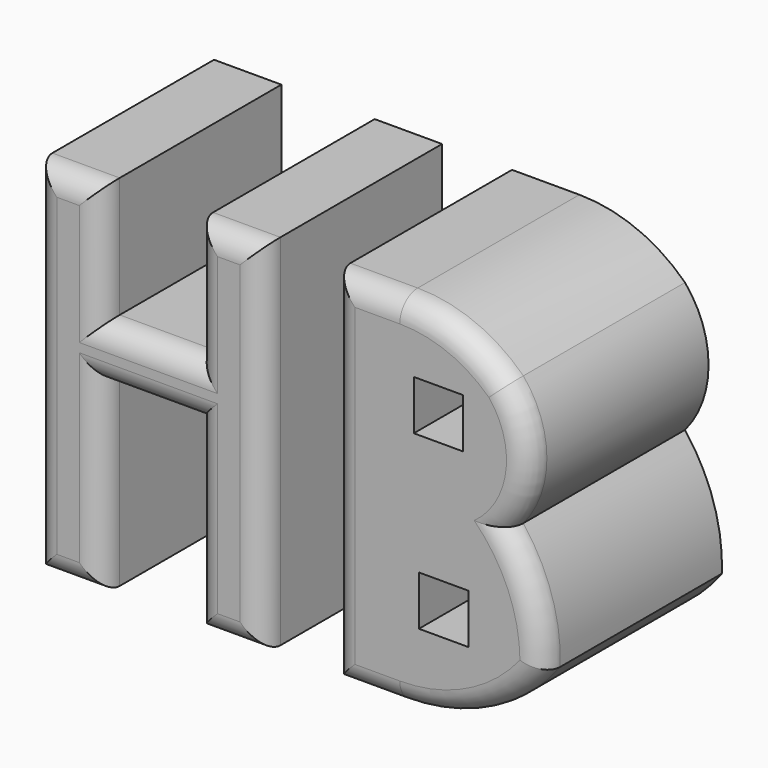
from build123d import *

# Parameters (mm, degrees)
F1_DEPTH       = 50
F0_W           = 11
F0_H           = 11.0476613045
F0_H_2         = 11.0476617701
F2_T1_DEPTH    = 105
F2_T3_DEPTH    = 40
F2_T5_DEPTH    = 39.3571444373
F2_T7_DEPTH    = 40
F2_T9_DEPTH    = 53.6428555627
F2_T11_DEPTH   = 20.7857115482
F2_T16_DEPTH   = 51.8571444373
F2_T21_DEPTH   = 66.1428555627
F2_T26_DEPTH   = 66.1428555627
F2_T31_DEPTH   = 51.8571444373
F2_T37_DEPTH   = 51.8571444373
F2_T42_DEPTH   = 33.2857115482
F2_T49_DEPTH   = 66.1428555627
F2_T54_DEPTH   = 33.2857115482
F2_T61_DEPTH   = 33.2857115482
F2_T65_DEPTH   = 66.1428555627
F2_T73_DEPTH   = 51.8571444373
F2_T78_DEPTH   = 33.2857115482
F2_2_T1_DEPTH  = 27.5
F2_2_T3_DEPTH  = 105
F2_2_T6_ANGLE  = 80.3342530923
F2_2_T10_ANGLE = 143.4118786012
F2_2_S11_R     = 39.2893999544
F2_2_T12_DEPTH = 27
F2_2_T16_ANGLE = 76.3206243735
F2_2_S17_R     = 22.5233307718
F2_2_T18_DEPTH = 29
F2_2_T20_ANGLE = 71.8308511896
F2_2_T25_ANGLE = 76.3206243735
F2_2_S26_R     = 22.5233307718
F2_2_T27_DEPTH = 29
F2_2_T30_ANGLE = 143.4118786012
F2_2_S31_R     = 39.2893999544
F2_2_T32_DEPTH = 27


# Not quite as in the source:
# - a fillet or chamfer that OpenCascade refuses, or shapes differently, is made with other operations: its cross-section is extruded or revolved along the edge and cut away or added


with BuildPart() as f1:
    # F0 (on Front) → F1 (new body)
    with BuildSketch(Plane.XZ):
        Polygon((-35.7857115482, 33.0714304233), (-50.7857115482, 33.0714304233), (-50.7857115482, -46.9285695767), (-35.7857115482, -46.9285695767), (-35.7857115482, -5.785714014), (-15, -5.785714014), (-15, -46.9285695767), (0, -46.9285695767), (0, 33.0714304233), (-15, 33.0714304233), (-15, 6.214285986), (-35.7857115482, 6.214285986), align=None)
    extrude(amount=F1_DEPTH)

    # F2: fillet of radius 5 on 12 edges, made by hand

    # F2_s2 → F2_t1 (cut)
    with BuildSketch(Plane.XY.offset(-59.4285695767)):
        with BuildLine():
            ThreePointArc((0, -45), (-1.4644660941, -48.5355339059), (-5, -50))
            Line((-5, -50), (0, -50))
            Line((0, -50), (0, -45))
        make_face()
        with BuildLine():
            ThreePointArc((-50.7857115482, -45), (-49.3212454541, -48.5355339059), (-45.7857115482, -50))
            Line((-45.7857115482, -50), (-50.7857115482, -50))
            Line((-50.7857115482, -50), (-50.7857115482, -45))
        make_face()
    extrude(amount=F2_T1_DEPTH, mode=Mode.SUBTRACT)

    # F2_s4 → F2_t3 (cut)
    with BuildSketch(Plane.YZ.offset(-27.5)):
        with BuildLine():
            ThreePointArc((-45, 33.0714304233), (-48.5355339059, 31.6069643292), (-50, 28.0714304233))
            Line((-50, 28.0714304233), (-50, 33.0714304233))
            Line((-50, 33.0714304233), (-45, 33.0714304233))
        make_face()
        with BuildLine():
            ThreePointArc((-45, -46.9285695767), (-48.5355339059, -45.4641034826), (-50, -41.9285695767))
            Line((-50, -41.9285695767), (-50, -46.9285695767))
            Line((-50, -46.9285695767), (-45, -46.9285695767))
        make_face()
    extrude(amount=F2_T3_DEPTH, mode=Mode.SUBTRACT)

    # F2_s6 → F2_t5 (cut)
    with BuildSketch(Plane.XY.offset(6.214285986)):
        with BuildLine():
            ThreePointArc((-35.7857115482, -45), (-37.2501776423, -48.5355339059), (-40.7857115482, -50))
            Line((-40.7857115482, -50), (-35.7857115482, -50))
            Line((-35.7857115482, -50), (-35.7857115482, -45))
        make_face()
        with BuildLine():
            ThreePointArc((-15, -45), (-13.5355339059, -48.5355339059), (-10, -50))
            Line((-10, -50), (-15, -50))
            Line((-15, -50), (-15, -45))
        make_face()
    extrude(amount=F2_T5_DEPTH, mode=Mode.SUBTRACT)

    # F2_s8 → F2_t7 (cut)
    with BuildSketch(Plane.YZ.offset(-63.2857115482)):
        with BuildLine():
            ThreePointArc((-45, 33.0714304233), (-48.5355339059, 31.6069643292), (-50, 28.0714304233))
            Line((-50, 28.0714304233), (-50, 33.0714304233))
            Line((-50, 33.0714304233), (-45, 33.0714304233))
        make_face()
        with BuildLine():
            ThreePointArc((-45, -46.9285695767), (-48.5355339059, -45.4641034826), (-50, -41.9285695767))
            Line((-50, -41.9285695767), (-50, -46.9285695767))
            Line((-50, -46.9285695767), (-45, -46.9285695767))
        make_face()
    extrude(amount=F2_T7_DEPTH, mode=Mode.SUBTRACT)

    # F2_s10 → F2_t9 (cut)
    with BuildSketch(Plane.XY.offset(-59.4285695767)):
        with BuildLine():
            ThreePointArc((-35.7857115482, -45), (-37.2501776423, -48.5355339059), (-40.7857115482, -50))
            Line((-40.7857115482, -50), (-35.7857115482, -50))
            Line((-35.7857115482, -50), (-35.7857115482, -45))
        make_face()
        with BuildLine():
            ThreePointArc((-15, -45), (-13.5355339059, -48.5355339059), (-10, -50))
            Line((-10, -50), (-15, -50))
            Line((-15, -50), (-15, -45))
        make_face()
    extrude(amount=F2_T9_DEPTH, mode=Mode.SUBTRACT)

    # F2_s12 → F2_t11 (cut)
    with BuildSketch(Plane.YZ.offset(-35.7857115482)):
        with BuildLine():
            ThreePointArc((-45, -5.785714014), (-48.5355339059, -4.3212479199), (-50, -0.785714014))
            Line((-50, -0.785714014), (-50, -5.785714014))
            Line((-50, -5.785714014), (-45, -5.785714014))
        make_face()
        with BuildLine():
            ThreePointArc((-45, 6.214285986), (-48.5355339059, 4.749819892), (-50, 1.214285986))
            Line((-50, 1.214285986), (-50, 6.214285986))
            Line((-50, 6.214285986), (-45, 6.214285986))
        make_face()
    extrude(amount=F2_T11_DEPTH, mode=Mode.SUBTRACT)


with BuildPart() as f1b:
    # F0 (on Front) → F1, piece 2 (new body)
    with BuildSketch(Plane.XZ):
        with BuildLine():
            Line((30.5800376087, 33.0714304233), (15.5800376087, 33.0714304233))
            Line((15.5800376087, 33.0714304233), (15.5800376087, -46.9285695767))
            Line((15.5800376087, -46.9285695767), (30.5800376087, -46.9285695767))
            ThreePointArc((30.5800376087, -46.9285695767), (48.3641167152, -42.6873971764), (62.3201467097, -30.8767985553))
            ThreePointArc((62.3201467097, -30.8767985553), (60.4523586567, -17.4078220357), (54.1052147746, -5.3821941838))
            ThreePointArc((54.1052147746, -5.3821941838), (59.3488970656, 9.0647493489), (54.1052147746, 23.5116928816))
            ThreePointArc((54.1052147746, 23.5116928816), (43.2767157427, 30.5902254056), (30.5800376087, 33.0714304233))
        make_face()
        with Locations((40.3426289856, -24.7864220291)):
            Rectangle(F0_W, F0_H, mode=Mode.SUBTRACT)
        with Locations((39.2095372379, 13.1722127553)):
            Rectangle(F0_W, F0_H_2, mode=Mode.SUBTRACT)
    extrude(amount=F1_DEPTH)

    # F2#2: fillet of radius 5 on 7 edges, made by hand

    # F2_2_s2 → F2_2_t1 (cut)
    with BuildSketch(Plane.YZ.offset(3.0800376087)):
        with BuildLine():
            ThreePointArc((-45, -46.9285695767), (-48.5355339059, -45.4641034826), (-50, -41.9285695767))
            Line((-50, -41.9285695767), (-50, -46.9285695767))
            Line((-50, -46.9285695767), (-45, -46.9285695767))
        make_face()
        with BuildLine():
            ThreePointArc((-45, 33.0714304233), (-48.5355339059, 31.6069643292), (-50, 28.0714304233))
            Line((-50, 28.0714304233), (-50, 33.0714304233))
            Line((-50, 33.0714304233), (-45, 33.0714304233))
        make_face()
    extrude(amount=F2_2_T1_DEPTH, mode=Mode.SUBTRACT)

    # F2_2_s4 → F2_2_t3 (cut)
    with BuildSketch(Plane.XY.offset(-59.4285695767)):
        with BuildLine():
            ThreePointArc((15.5800376087, -45), (17.0445037028, -48.5355339059), (20.5800376087, -50))
            Line((20.5800376087, -50), (15.5800376087, -50))
            Line((15.5800376087, -50), (15.5800376087, -45))
        make_face()
    extrude(amount=F2_2_T3_DEPTH, mode=Mode.SUBTRACT)

    # F2_2_s5 → F2_2_t6 (revolve, cut)
    with BuildSketch(Plane(origin=(0.9703990257, 0, -5.6975752164), x_dir=(0, 1, 0), z_dir=(0.1679000671, 0, -0.9858040208))):
        with BuildLine():
            ThreePointArc((-45, 63.7619837133), (-48.5355339059, 62.2975176192), (-50, 58.7619837133))
            Line((-50, 58.7619837133), (-50, 63.7619837133))
            Line((-50, 63.7619837133), (-45, 63.7619837133))
        make_face()
    revolve(axis=Axis((30.5800376087, -50, -0.6545238583), (0, -1, 0)), revolution_arc=F2_2_T6_ANGLE, mode=Mode.SUBTRACT)


with BuildPart() as f2_tool14:
    # F2_s15 → F2_t16 (new body)
    with BuildSketch(Plane.XY.offset(-6.285714014)):
        with BuildLine():
            ThreePointArc((-35.7857115482, -45), (-37.2501776423, -48.5355339059), (-40.7857115482, -50))
            Line((-40.7857115482, -50), (-35.7857115482, -50))
            Line((-35.7857115482, -50), (-35.7857115482, -45))
        make_face()
    extrude(amount=F2_T16_DEPTH)

    split(bisect_by=Plane.XY.offset(-5.785714014), keep=Keep.BOTTOM)


with BuildPart() as f1_1:
    add(f1.part)

    # F2_t13: cut F2_tool14
    add(f2_tool14.part, mode=Mode.SUBTRACT)


with BuildPart() as f2_tool19:
    # F2_s20 → F2_t21 (new body)
    with BuildSketch(Plane.XY.offset(-59.4285695767)):
        with BuildLine():
            ThreePointArc((-35.7857115482, -45), (-37.2501776423, -48.5355339059), (-40.7857115482, -50))
            Line((-40.7857115482, -50), (-35.7857115482, -50))
            Line((-35.7857115482, -50), (-35.7857115482, -45))
        make_face()
    extrude(amount=F2_T21_DEPTH)

    split(bisect_by=Plane.XY.offset(6.214285986), keep=Keep.TOP)


with BuildPart() as f1_2:
    add(f1_1.part)

    # F2_t18: cut F2_tool19
    add(f2_tool19.part, mode=Mode.SUBTRACT)


with BuildPart() as f2_tool24:
    # F2_s25 → F2_t26 (new body)
    with BuildSketch(Plane.XY.offset(6.714285986)):
        with BuildLine():
            ThreePointArc((-15, -45), (-13.5355339059, -48.5355339059), (-10, -50))
            Line((-10, -50), (-15, -50))
            Line((-15, -50), (-15, -45))
        make_face()
    extrude(amount=-F2_T26_DEPTH)

    split(bisect_by=Plane.XY.offset(6.214285986), keep=Keep.TOP)


with BuildPart() as f1_3:
    add(f1_2.part)

    # F2_t23: cut F2_tool24
    add(f2_tool24.part, mode=Mode.SUBTRACT)


with BuildPart() as f2_tool29:
    # F2_s30 → F2_t31 (new body)
    with BuildSketch(Plane.XY.offset(45.5714304233)):
        with BuildLine():
            ThreePointArc((-15, -45), (-13.5355339059, -48.5355339059), (-10, -50))
            Line((-10, -50), (-15, -50))
            Line((-15, -50), (-15, -45))
        make_face()
    extrude(amount=-F2_T31_DEPTH)

    split(bisect_by=Plane.XY.offset(-5.785714014), keep=Keep.BOTTOM)


with BuildPart() as f1_4:
    add(f1_3.part)

    # F2_t28: cut F2_tool29
    add(f2_tool29.part, mode=Mode.SUBTRACT)


with BuildPart() as f2_tool35:
    # F2_s36 → F2_t37 (new body)
    with BuildSketch(Plane.XY.offset(-6.285714014)):
        with BuildLine():
            ThreePointArc((-35.7857115482, -45), (-37.2501776423, -48.5355339059), (-40.7857115482, -50))
            Line((-40.7857115482, -50), (-35.7857115482, -50))
            Line((-35.7857115482, -50), (-35.7857115482, -45))
        make_face()
    extrude(amount=F2_T37_DEPTH)

    split(bisect_by=Plane.XY.offset(6.214285986), keep=Keep.BOTTOM)

    split(bisect_by=Plane.XY.offset(-5.785714014), keep=Keep.TOP)


with BuildPart() as f2_tool40:
    # F2_s41 → F2_t42 (new body)
    with BuildSketch(Plane.YZ.offset(-15)):
        with BuildLine():
            ThreePointArc((-45, 6.214285986), (-48.5355339059, 4.749819892), (-50, 1.214285986))
            Line((-50, 1.214285986), (-50, 6.214285986))
            Line((-50, 6.214285986), (-45, 6.214285986))
        make_face()
    extrude(amount=-F2_T42_DEPTH)

    split(bisect_by=Plane.YZ.offset(-35.7857115482), keep=Keep.BOTTOM)


with BuildPart() as f2_tool35_1:
    add(f2_tool35.part)

    # F2_t44: intersect F2_tool40
    add(f2_tool40.part, mode=Mode.INTERSECT)


with BuildPart() as f1_5:
    add(f1_4.part)

    # F2_t33: cut F2_tool35
    add(f2_tool35_1.part, mode=Mode.SUBTRACT)


with BuildPart() as f2_tool47:
    # F2_s48 → F2_t49 (new body)
    with BuildSketch(Plane.XY.offset(-59.4285695767)):
        with BuildLine():
            ThreePointArc((-35.7857115482, -45), (-37.2501776423, -48.5355339059), (-40.7857115482, -50))
            Line((-40.7857115482, -50), (-35.7857115482, -50))
            Line((-35.7857115482, -50), (-35.7857115482, -45))
        make_face()
    extrude(amount=F2_T49_DEPTH)

    split(bisect_by=Plane.XY.offset(6.214285986), keep=Keep.BOTTOM)

    split(bisect_by=Plane.XY.offset(-5.785714014), keep=Keep.TOP)


with BuildPart() as f2_tool52:
    # F2_s53 → F2_t54 (new body)
    with BuildSketch(Plane.YZ.offset(-48.2857115482)):
        with BuildLine():
            ThreePointArc((-45, -5.785714014), (-48.5355339059, -4.3212479199), (-50, -0.785714014))
            Line((-50, -0.785714014), (-50, -5.785714014))
            Line((-50, -5.785714014), (-45, -5.785714014))
        make_face()
    extrude(amount=F2_T54_DEPTH)

    split(bisect_by=Plane.YZ.offset(-35.7857115482), keep=Keep.BOTTOM)


with BuildPart() as f2_tool47_1:
    add(f2_tool47.part)

    # F2_t56: intersect F2_tool52
    add(f2_tool52.part, mode=Mode.INTERSECT)


with BuildPart() as f1_6:
    add(f1_5.part)

    # F2_t45: cut F2_tool47
    add(f2_tool47_1.part, mode=Mode.SUBTRACT)


with BuildPart() as f2_tool59:
    # F2_s60 → F2_t61 (new body)
    with BuildSketch(Plane.YZ.offset(-35.7857115482)):
        with BuildLine():
            ThreePointArc((-45, -5.785714014), (-48.5355339059, -4.3212479199), (-50, -0.785714014))
            Line((-50, -0.785714014), (-50, -5.785714014))
            Line((-50, -5.785714014), (-45, -5.785714014))
        make_face()
    extrude(amount=F2_T61_DEPTH)

    split(bisect_by=Plane.YZ.offset(-15), keep=Keep.TOP)


with BuildPart() as f2_tool63:
    # F2_s64 → F2_t65 (new body)
    with BuildSketch(Plane.XY.offset(6.714285986)):
        with BuildLine():
            ThreePointArc((-15, -45), (-13.5355339059, -48.5355339059), (-10, -50))
            Line((-10, -50), (-15, -50))
            Line((-15, -50), (-15, -45))
        make_face()
    extrude(amount=-F2_T65_DEPTH)

    split(bisect_by=Plane.XY.offset(-5.785714014), keep=Keep.TOP)

    split(bisect_by=Plane.XY.offset(6.214285986), keep=Keep.BOTTOM)


with BuildPart() as f2_tool59_1:
    add(f2_tool59.part)

    # F2_t68: intersect F2_tool63
    add(f2_tool63.part, mode=Mode.INTERSECT)


with BuildPart() as f1_7:
    add(f1_6.part)

    # F2_t57: cut F2_tool59
    add(f2_tool59_1.part, mode=Mode.SUBTRACT)


with BuildPart() as f2_tool71:
    # F2_s72 → F2_t73 (new body)
    with BuildSketch(Plane.XY.offset(45.5714304233)):
        with BuildLine():
            ThreePointArc((-15, -45), (-13.5355339059, -48.5355339059), (-10, -50))
            Line((-10, -50), (-15, -50))
            Line((-15, -50), (-15, -45))
        make_face()
    extrude(amount=-F2_T73_DEPTH)

    split(bisect_by=Plane.XY.offset(-5.785714014), keep=Keep.TOP)

    split(bisect_by=Plane.XY.offset(6.214285986), keep=Keep.BOTTOM)


with BuildPart() as f2_tool76:
    # F2_s77 → F2_t78 (new body)
    with BuildSketch(Plane.YZ.offset(-2.5)):
        with BuildLine():
            ThreePointArc((-45, 6.214285986), (-48.5355339059, 4.749819892), (-50, 1.214285986))
            Line((-50, 1.214285986), (-50, 6.214285986))
            Line((-50, 6.214285986), (-45, 6.214285986))
        make_face()
    extrude(amount=-F2_T78_DEPTH)

    split(bisect_by=Plane.YZ.offset(-15), keep=Keep.TOP)


with BuildPart() as f2_tool71_1:
    add(f2_tool71.part)

    # F2_t80: intersect F2_tool76
    add(f2_tool76.part, mode=Mode.INTERSECT)


with BuildPart() as f1_8:
    add(f1_7.part)

    # F2_t69: cut F2_tool71
    add(f2_tool71_1.part, mode=Mode.SUBTRACT)


with BuildPart() as f2_2_tool8:
    # F2_2_s9 → F2_2_t10 (revolve)
    with BuildSketch(Plane(origin=(35.8987230001, 0, 11.8682393716), x_dir=(0, 1, 0), z_dir=(-0.9494580211, 0, -0.3138940365))):
        with BuildLine():
            ThreePointArc((-45, 25.4760574436), (-48.5355339059, 24.0115913495), (-50, 20.4760574436))
            Line((-50, 20.4760574436), (-50, 25.4760574436))
            Line((-50, 25.4760574436), (-45, 25.4760574436))
        make_face()
    revolve(axis=Axis((36.8255662938, -50, 9.0647493489), (0, -1, 0)), revolution_arc=F2_2_T10_ANGLE)

    # F2_2_s11 → F2_2_t12 (cut, symmetric)
    with BuildSketch(Plane.XZ.offset(47.5)):
        with Locations((23.056385538, -29.4576412578)):
            Circle(F2_2_S11_R)
    extrude(amount=F2_2_T12_DEPTH, both=True, mode=Mode.SUBTRACT)


with BuildPart() as f1b_1:
    add(f1b.part)

    # F2_2_t7: cut F2_2_tool8
    add(f2_2_tool8.part, mode=Mode.SUBTRACT)


with BuildPart() as f2_2_tool14:
    # F2_2_s15 → F2_2_t16 (revolve)
    with BuildSketch(Plane(origin=(-6.8099969571, 0, -18.4096063069), x_dir=(0, 1, 0), z_dir=(-0.3469390933, 0, -0.9378876615))):
        with BuildLine():
            ThreePointArc((-45, 71.133706818), (-48.5355339059, 69.669240724), (-50, 66.133706818))
            Line((-50, 66.133706818), (-50, 71.133706818))
            Line((-50, 71.133706818), (-45, 71.133706818))
        make_face()
    revolve(axis=Axis((23.056385538, -50, -29.4576412578), (0, -1, 0)), revolution_arc=F2_2_T16_ANGLE)

    # F2_2_s17 → F2_2_t18 (cut, symmetric)
    with BuildSketch(Plane.XZ.offset(47.5)):
        with Locations((36.8255662938, 9.0647493489)):
            Circle(F2_2_S17_R)
    extrude(amount=F2_2_T18_DEPTH, both=True, mode=Mode.SUBTRACT)


with BuildPart() as f1b_2:
    add(f1b_1.part)

    # F2_2_t13: cut F2_2_tool14
    add(f2_2_tool14.part, mode=Mode.SUBTRACT)

    # F2_2_s19 → F2_2_t20 (revolve, cut)
    with BuildSketch(Plane.YZ.offset(30.5800376087)):
        with BuildLine():
            ThreePointArc((-45, -46.9285695767), (-48.5355339059, -45.4641034826), (-50, -41.9285695767))
            Line((-50, -41.9285695767), (-50, -46.9285695767))
            Line((-50, -46.9285695767), (-45, -46.9285695767))
        make_face()
    revolve(axis=Axis((30.5800376087, -50, -7.5218936101), (0, -1, 0)), revolution_arc=F2_2_T20_ANGLE, mode=Mode.SUBTRACT)


with BuildPart() as f2_2_tool23:
    # F2_2_s24 → F2_2_t25 (revolve)
    with BuildSketch(Plane(origin=(-6.8099969571, 0, -18.4096063069), x_dir=(0, 1, 0), z_dir=(-0.3469390933, 0, -0.9378876615))):
        with BuildLine():
            ThreePointArc((-45, 71.133706818), (-48.5355339059, 69.669240724), (-50, 66.133706818))
            Line((-50, 66.133706818), (-50, 71.133706818))
            Line((-50, 71.133706818), (-45, 71.133706818))
        make_face()
    revolve(axis=Axis((23.056385538, -50, -29.4576412578), (0, -1, 0)), revolution_arc=F2_2_T25_ANGLE)

    # F2_2_s26 → F2_2_t27 (intersect, symmetric)
    with BuildSketch(Plane.XZ.offset(47.5)):
        with Locations((36.8255662938, 9.0647493489)):
            Circle(F2_2_S26_R)
    extrude(amount=F2_2_T27_DEPTH, both=True, mode=Mode.INTERSECT)


with BuildPart() as f2_2_tool28:
    # F2_2_s29 → F2_2_t30 (revolve)
    with BuildSketch(Plane(origin=(35.8987230001, 0, 11.8682393716), x_dir=(0, 1, 0), z_dir=(-0.9494580211, 0, -0.3138940365))):
        with BuildLine():
            ThreePointArc((-45, 25.4760574436), (-48.5355339059, 24.0115913495), (-50, 20.4760574436))
            Line((-50, 20.4760574436), (-50, 25.4760574436))
            Line((-50, 25.4760574436), (-45, 25.4760574436))
        make_face()
    revolve(axis=Axis((36.8255662938, -50, 9.0647493489), (0, -1, 0)), revolution_arc=F2_2_T30_ANGLE)

    # F2_2_s31 → F2_2_t32 (intersect, symmetric)
    with BuildSketch(Plane.XZ.offset(47.5)):
        with Locations((23.056385538, -29.4576412578)):
            Circle(F2_2_S31_R)
    extrude(amount=F2_2_T32_DEPTH, both=True, mode=Mode.INTERSECT)


with BuildPart() as f2_2_tool23_1:
    add(f2_2_tool23.part)

    # F2_2_t33: intersect F2_2_tool28
    add(f2_2_tool28.part, mode=Mode.INTERSECT)


with BuildPart() as f1b_3:
    add(f1b_2.part)

    # F2_2_t21: cut F2_2_tool23
    add(f2_2_tool23_1.part, mode=Mode.SUBTRACT)


solid = Compound([f1_8.part, f1b_3.part])
